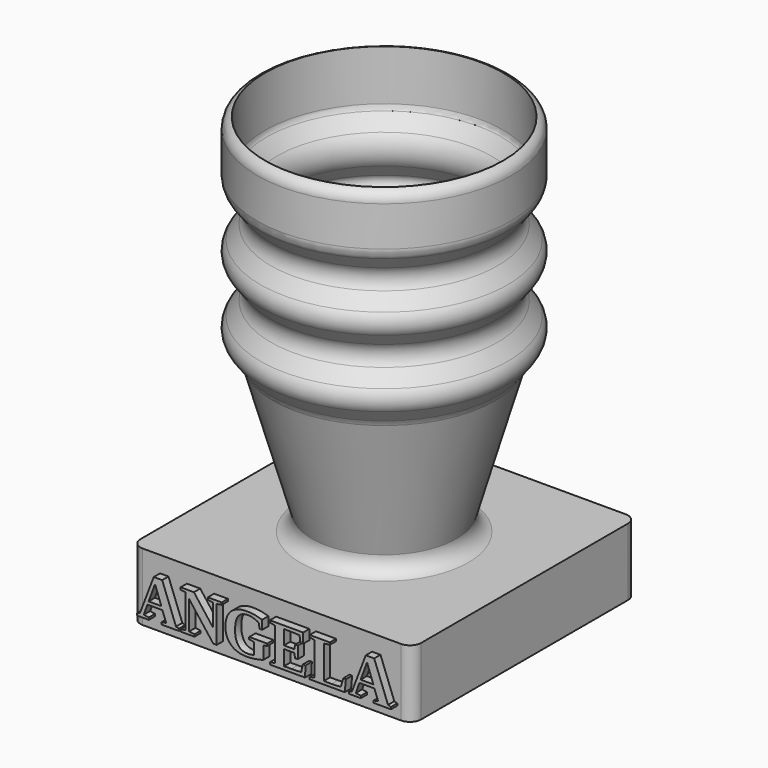
from build123d import *

# Parameters (mm, degrees)
F0_W         = 50
F0_H         = 50
F1_DEPTH     = 12
F2_TEXT_SIZE = 10.6147467099
F3_DEPTH     = 1.4
F4_R         = 2
F7_T         = -1.4
F9_R         = 4.5
F9_R_2       = 3.5
F10_DEPTH    = 5
F11_T        = 2


# Not quite as in the source:
# - a fillet or chamfer that OpenCascade refuses, or shapes differently, is made with other operations: its cross-section is extruded or revolved along the edge and cut away or added
# - a shell that OpenCascade refuses in one call is made with other operations: the cavity is built on its own and cut out
# - Text() gives the source's letters only with a copy of the font that has no kerning and outlines rounded to 1/6400 em; it was checked with that copy


with BuildPart() as f1:
    # F0 (on Top) → F1 (new body)
    with BuildSketch(Plane.XY):
        Rectangle(F0_W, F0_H)
    extrude(amount=F1_DEPTH)

    # F4
    f4_edges = [f1.edges().sort_by_distance(p)[0] for p in [
        (-25, -25, 6),
        (-25, 25, 6),
        (25, -25, 6),
        (25, 25, 6),
    ]]
    fillet(f4_edges, radius=F4_R)

    # F11: shell of thickness 2, made by hand


with BuildPart() as f3:
    # F2 (on face) → F3 (new body)
    with BuildSketch(Plane.XZ.offset(25)):
        with Locations((-23, 2.1)):
            Text('ANGELA', F2_TEXT_SIZE, font='Tinos', font_style=FontStyle.BOLD, text_align=(TextAlign.LEFT, TextAlign.BOTTOM))
    extrude(amount=F3_DEPTH)


with BuildPart() as f6:
    # F5 (on Front) → F6 (revolve)
    with BuildSketch(Plane.XZ):
        with BuildLine():
            Line((0, 12), (0, 77))
            Line((0, 77), (-22.6, 77))
            Line((-22.6, 77), (-22.6, 68))
            ThreePointArc((-22.6, 68), (-22.4460498942, 67.0513167019), (-22, 66.2))
            Line((-22, 66.2), (-20.2, 63.8))
            ThreePointArc((-20.2, 63.8), (-19.6, 62), (-20.2, 60.2))
            Line((-20.2, 60.2), (-22, 57.8))
            ThreePointArc((-22, 57.8), (-22.6, 56), (-22, 54.2))
            Line((-22, 54.2), (-20.2, 51.8))
            ThreePointArc((-20.2, 51.8), (-19.6, 50), (-20.2, 48.2))
            Line((-20.2, 48.2), (-22, 45.8))
            ThreePointArc((-22, 45.8), (-22.6, 44), (-22, 42.2))
            Line((-22, 42.2), (-20.2, 39.8))
            ThreePointArc((-20.2, 39.8), (-19.914224551, 39.3366414021), (-19.7168913288, 38.8292673814))
            Line((-19.7168913288, 38.8292673814), (-12.862888787, 15))
            ThreePointArc((-12.862888787, 15), (-13.4168304928, 13.1334042875), (-15, 12))
            Line((-15, 12), (-12, 12))
            Line((-12, 12), (0, 12))
        make_face()
    revolve(axis=Axis((0, 0, 44.5), (0, 0, -1)))

    # F7
    f7_openings = [f6.faces().sort_by_distance(p)[0] for p in [
        (0, 0, 77),
    ]]
    offset(amount=F7_T, openings=f7_openings, kind=Kind.INTERSECTION)

    # F8: fillet of radius 2 on 1 edges, made by hand

    # F8_s1 → F8_t2 (revolve, cut)
    with BuildSketch(Plane.XZ):
        with BuildLine():
            ThreePointArc((-22.6, 75.0921215972), (-22.2124515497, 76.2753375538), (-21.2, 77))
            Line((-21.2, 77), (-22.6, 77))
            Line((-22.6, 77), (-22.6, 75.0921215972))
        make_face()
    revolve(axis=Axis((0, 0, 77), (0, 0, -1)), mode=Mode.SUBTRACT)


with BuildPart() as f10:
    # F9 (on face) → F10 (new body)
    with BuildSketch(Plane.XY.offset(13.4)):
        Circle(F9_R)
        Circle(F9_R_2, mode=Mode.SUBTRACT)
    extrude(amount=F10_DEPTH)


with BuildPart() as f11_core1:
    # F11_t2: copy of F1
    add(f1.part)

    # the walls: a layer under each face that stays
    f11_faces = [f11_core1.faces().sort_by_distance(p)[0] for p in [
        (25, 0, 6),
        (0, 0, 0),
        (0, 0, 12),
        (0, -25, 6),
        (0, 25, 6),
        (-25, 0, 6),
    ]]
    thicken(f11_faces, amount=-F11_T, mode=Mode.SUBTRACT)


with BuildPart() as f1_1:
    add(f1.part)

    # what is left inside the walls is the cavity
    f11_cavity = [f11_core1.part.solids().sort_by_distance(p)[0] for p in [
        (0, -7.666667, 2.02),
    ]]
    add(f11_cavity, mode=Mode.SUBTRACT)


solid = Compound([f3.part, f6.part, f10.part, f1_1.part])
